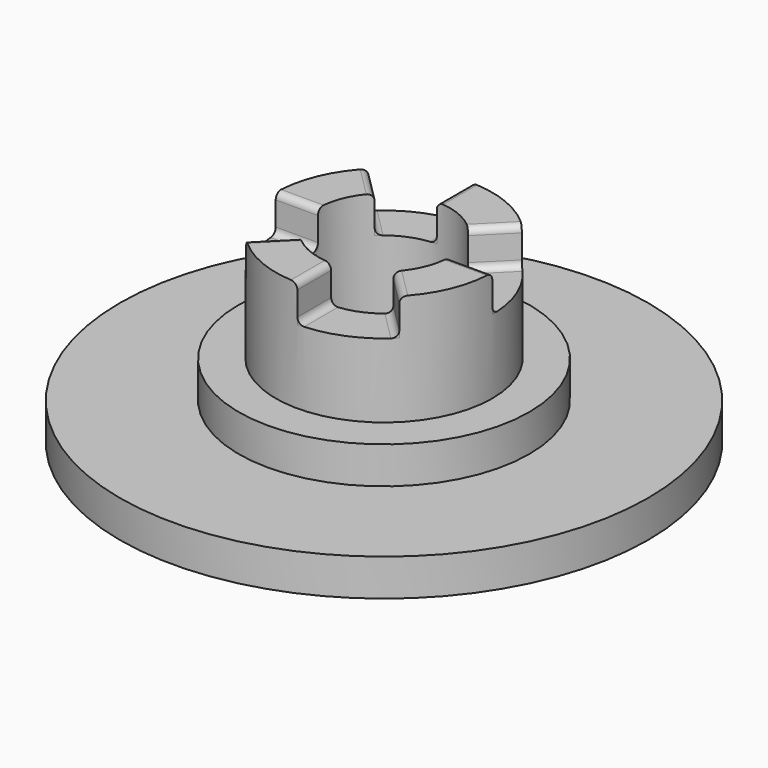
from build123d import *

# Parameters (mm, degrees)
F0_R         = 10
F1_DEPTH     = 1.4
F2_R         = 5.5
F3_DEPTH     = 1.4
F4_R         = 4.1
F4_R_2       = 2.5
F5_DEPTH     = 4.2
F7_DEPTH     = 1.4
F8_T4_DEPTH  = 2.85
F8_S5_R      = 4.1
F8_T6_DEPTH  = 3
F8_S7_R      = 2.5
F8_T8_DEPTH  = 3
F8_T12_DEPTH = 2.85
F8_S13_R     = 4.1
F8_T14_DEPTH = 3
F8_S15_R     = 2.5
F8_T16_DEPTH = 3
F8_T20_DEPTH = 2.85
F8_S21_R     = 4.1
F8_T22_DEPTH = 3
F8_S23_R     = 2.5
F8_T24_DEPTH = 3
F8_T28_DEPTH = 2.85
F8_S29_R     = 4.1
F8_T30_DEPTH = 3
F8_S31_R     = 2.5
F8_T32_DEPTH = 3
F8_T36_DEPTH = 2.85
F8_S37_R     = 4.1
F8_T38_DEPTH = 3
F8_S39_R     = 2.5
F8_T40_DEPTH = 3
F8_T44_DEPTH = 2.85
F8_S45_R     = 4.1
F8_T46_DEPTH = 3
F8_S47_R     = 2.5
F8_T48_DEPTH = 3
F8_T52_DEPTH = 2.85
F8_S53_R     = 4.1
F8_T54_DEPTH = 3
F8_S55_R     = 2.5
F8_T56_DEPTH = 3
F8_T60_DEPTH = 2.85
F8_S61_R     = 4.1
F8_T62_DEPTH = 3
F8_S63_R     = 2.5
F8_T64_DEPTH = 3
F8_T65_DEPTH = 2.85
F8_T67_DEPTH = 2.85
F8_T69_DEPTH = 2.85
F8_T71_DEPTH = 2.85
F8_T73_DEPTH = 2.85
F8_T75_DEPTH = 2.85
F8_T77_DEPTH = 2.85
F8_T79_DEPTH = 2.85


# Not quite as in the source:
# - a fillet or chamfer that OpenCascade refuses, or shapes differently, is made with other operations: its cross-section is extruded or revolved along the edge and cut away or added


with BuildPart() as f1:
    # F0 (on Top) → F1 (new body)
    with BuildSketch(Plane.XY):
        Circle(F0_R)
    extrude(amount=F1_DEPTH)

    # F2 (on face) → F3 (join)
    with BuildSketch(Plane.XY.offset(1.4)):
        Circle(F2_R)
    extrude(amount=F3_DEPTH)

    # F4 (on face) → F5 (join)
    with BuildSketch(Plane.XY.offset(2.8)):
        Circle(F4_R)
        Circle(F4_R_2, mode=Mode.SUBTRACT)
    extrude(amount=F5_DEPTH)

    # F6 (on face) → F7 (cut)
    with BuildSketch(Plane.XY.offset(7)):
        with BuildLine():
            Line((0, -2.5), (0, -4.1))
            ThreePointArc((0, -4.1), (1.5690020727, -3.7879060833), (2.8991378029, -2.8991378029))
            Line((2.8991378029, -2.8991378029), (1.767766953, -1.767766953))
            ThreePointArc((1.767766953, -1.767766953), (0.9567085809, -2.3096988313), (0, -2.5))
        make_face()
        with BuildLine():
            ThreePointArc((-4.1, 0), (-3.7879060833, -1.5690020727), (-2.8991378029, -2.8991378029))
            Line((-2.8991378029, -2.8991378029), (-1.767766953, -1.767766953))
            ThreePointArc((-1.767766953, -1.767766953), (-2.3096988313, -0.9567085809), (-2.5, 0))
            Line((-2.5, 0), (-4.1, 0))
        make_face()
        with BuildLine():
            Line((2.5, 0), (4.1, 0))
            ThreePointArc((4.1, 0), (3.7879060833, 1.5690020727), (2.8991378029, 2.8991378029))
            Line((2.8991378029, 2.8991378029), (1.767766953, 1.767766953))
            ThreePointArc((1.767766953, 1.767766953), (2.3096988313, 0.9567085809), (2.5, 0))
        make_face()
        with BuildLine():
            ThreePointArc((-1.767766953, 1.767766953), (-0.9567085809, 2.3096988313), (0, 2.5))
            Line((0, 2.5), (0, 4.1))
            ThreePointArc((0, 4.1), (-1.5690020727, 3.7879060833), (-2.8991378029, 2.8991378029))
            Line((-2.8991378029, 2.8991378029), (-1.767766953, 1.767766953))
        make_face()
    extrude(amount=-F7_DEPTH, mode=Mode.SUBTRACT)

    # F8: fillet of radius 0.25 on 16 edges, made by hand


with BuildPart() as f8_tool2:
    # F8_s3 → F8_t4 (new body)
    with BuildSketch(Plane.YZ.offset(-1.875)):
        with BuildLine():
            ThreePointArc((-0.25, 5.6), (-0.0732233047, 5.6732233047), (0, 5.85))
            Line((0, 5.85), (0, 5.6))
            Line((0, 5.6), (-0.25, 5.6))
        make_face()
    extrude(amount=-F8_T4_DEPTH)

    # F8_s5 → F8_t6 (intersect, symmetric)
    with BuildSketch(Plane.XY.offset(5.7)):
        Circle(F8_S5_R)
    extrude(amount=F8_T6_DEPTH, both=True, mode=Mode.INTERSECT)

    # F8_s7 → F8_t8 (cut, symmetric)
    with BuildSketch(Plane.XY.offset(5.7)):
        Circle(F8_S7_R)
    extrude(amount=F8_T8_DEPTH, both=True, mode=Mode.SUBTRACT)


with BuildPart() as f1_1:
    add(f1.part)

    # F8_t1: union F8_tool2
    add(f8_tool2.part)


with BuildPart() as f8_tool10:
    # F8_s11 → F8_t12 (new body)
    with BuildSketch(Plane.XZ.offset(-1.875)):
        with BuildLine():
            ThreePointArc((-0.25, 5.6), (-0.0732233047, 5.6732233047), (0, 5.85))
            Line((0, 5.85), (0, 5.6))
            Line((0, 5.6), (-0.25, 5.6))
        make_face()
    extrude(amount=-F8_T12_DEPTH)

    # F8_s13 → F8_t14 (intersect, symmetric)
    with BuildSketch(Plane.XY.offset(5.7)):
        Circle(F8_S13_R)
    extrude(amount=F8_T14_DEPTH, both=True, mode=Mode.INTERSECT)

    # F8_s15 → F8_t16 (cut, symmetric)
    with BuildSketch(Plane.XY.offset(5.7)):
        Circle(F8_S15_R)
    extrude(amount=F8_T16_DEPTH, both=True, mode=Mode.SUBTRACT)


with BuildPart() as f1_2:
    add(f1_1.part)

    # F8_t9: union F8_tool10
    add(f8_tool10.part)


with BuildPart() as f8_tool18:
    # F8_s19 → F8_t20 (new body)
    with BuildSketch(Plane(origin=(3.3410795411, -3.3410795411, 0), x_dir=(0, 0, 1), z_dir=(-0.7071067812, 0.7071067812, 0))):
        with BuildLine():
            ThreePointArc((5.85, 0), (5.6732233047, -0.0732233047), (5.6, -0.25))
            Line((5.6, -0.25), (5.6, 0))
            Line((5.6, 0), (5.85, 0))
        make_face()
    extrude(amount=F8_T20_DEPTH)

    # F8_s21 → F8_t22 (intersect, symmetric)
    with BuildSketch(Plane.XY.offset(5.7)):
        Circle(F8_S21_R)
    extrude(amount=F8_T22_DEPTH, both=True, mode=Mode.INTERSECT)

    # F8_s23 → F8_t24 (cut, symmetric)
    with BuildSketch(Plane.XY.offset(5.7)):
        Circle(F8_S23_R)
    extrude(amount=F8_T24_DEPTH, both=True, mode=Mode.SUBTRACT)


with BuildPart() as f1_3:
    add(f1_2.part)

    # F8_t17: union F8_tool18
    add(f8_tool18.part)


with BuildPart() as f8_tool26:
    # F8_s27 → F8_t28 (new body)
    with BuildSketch(Plane.YZ.offset(1.875)):
        with BuildLine():
            ThreePointArc((0, 5.85), (0.0732233047, 5.6732233047), (0.25, 5.6))
            Line((0.25, 5.6), (0, 5.6))
            Line((0, 5.6), (0, 5.85))
        make_face()
    extrude(amount=F8_T28_DEPTH)

    # F8_s29 → F8_t30 (intersect, symmetric)
    with BuildSketch(Plane.XY.offset(5.7)):
        Circle(F8_S29_R)
    extrude(amount=F8_T30_DEPTH, both=True, mode=Mode.INTERSECT)

    # F8_s31 → F8_t32 (cut, symmetric)
    with BuildSketch(Plane.XY.offset(5.7)):
        Circle(F8_S31_R)
    extrude(amount=F8_T32_DEPTH, both=True, mode=Mode.SUBTRACT)


with BuildPart() as f1_4:
    add(f1_3.part)

    # F8_t25: union F8_tool26
    add(f8_tool26.part)


with BuildPart() as f8_tool34:
    # F8_s35 → F8_t36 (new body)
    with BuildSketch(Plane(origin=(-3.3410795411, -3.3410795411, 0), x_dir=(0, 0, 1), z_dir=(0.7071067812, 0.7071067812, 0))):
        with BuildLine():
            ThreePointArc((5.85, 0), (5.6732233047, -0.0732233047), (5.6, -0.25))
            Line((5.6, -0.25), (5.6, 0))
            Line((5.6, 0), (5.85, 0))
        make_face()
    extrude(amount=F8_T36_DEPTH)

    # F8_s37 → F8_t38 (intersect, symmetric)
    with BuildSketch(Plane.XY.offset(5.7)):
        Circle(F8_S37_R)
    extrude(amount=F8_T38_DEPTH, both=True, mode=Mode.INTERSECT)

    # F8_s39 → F8_t40 (cut, symmetric)
    with BuildSketch(Plane.XY.offset(5.7)):
        Circle(F8_S39_R)
    extrude(amount=F8_T40_DEPTH, both=True, mode=Mode.SUBTRACT)


with BuildPart() as f1_5:
    add(f1_4.part)

    # F8_t33: union F8_tool34
    add(f8_tool34.part)


with BuildPart() as f8_tool42:
    # F8_s43 → F8_t44 (new body)
    with BuildSketch(Plane(origin=(-3.3410795411, 3.3410795411, 0), x_dir=(0, 0, 1), z_dir=(0.7071067812, -0.7071067812, 0))):
        with BuildLine():
            ThreePointArc((5.85, 0), (5.6732233047, -0.0732233047), (5.6, -0.25))
            Line((5.6, -0.25), (5.6, 0))
            Line((5.6, 0), (5.85, 0))
        make_face()
    extrude(amount=F8_T44_DEPTH)

    # F8_s45 → F8_t46 (intersect, symmetric)
    with BuildSketch(Plane.XY.offset(5.7)):
        Circle(F8_S45_R)
    extrude(amount=F8_T46_DEPTH, both=True, mode=Mode.INTERSECT)

    # F8_s47 → F8_t48 (cut, symmetric)
    with BuildSketch(Plane.XY.offset(5.7)):
        Circle(F8_S47_R)
    extrude(amount=F8_T48_DEPTH, both=True, mode=Mode.SUBTRACT)


with BuildPart() as f1_6:
    add(f1_5.part)

    # F8_t41: union F8_tool42
    add(f8_tool42.part)


with BuildPart() as f8_tool50:
    # F8_s51 → F8_t52 (new body)
    with BuildSketch(Plane.XZ.offset(1.875)):
        with BuildLine():
            ThreePointArc((0.25, 5.6), (0.0732233047, 5.6732233047), (0, 5.85))
            Line((0, 5.85), (0, 5.6))
            Line((0, 5.6), (0.25, 5.6))
        make_face()
    extrude(amount=F8_T52_DEPTH)

    # F8_s53 → F8_t54 (intersect, symmetric)
    with BuildSketch(Plane.XY.offset(5.7)):
        Circle(F8_S53_R)
    extrude(amount=F8_T54_DEPTH, both=True, mode=Mode.INTERSECT)

    # F8_s55 → F8_t56 (cut, symmetric)
    with BuildSketch(Plane.XY.offset(5.7)):
        Circle(F8_S55_R)
    extrude(amount=F8_T56_DEPTH, both=True, mode=Mode.SUBTRACT)


with BuildPart() as f1_7:
    add(f1_6.part)

    # F8_t49: union F8_tool50
    add(f8_tool50.part)


with BuildPart() as f8_tool58:
    # F8_s59 → F8_t60 (new body)
    with BuildSketch(Plane(origin=(3.3410795411, 3.3410795411, 0), x_dir=(0, 0, 1), z_dir=(-0.7071067812, -0.7071067812, 0))):
        with BuildLine():
            ThreePointArc((5.85, 0), (5.6732233047, -0.0732233047), (5.6, -0.25))
            Line((5.6, -0.25), (5.6, 0))
            Line((5.6, 0), (5.85, 0))
        make_face()
    extrude(amount=F8_T60_DEPTH)

    # F8_s61 → F8_t62 (intersect, symmetric)
    with BuildSketch(Plane.XY.offset(5.7)):
        Circle(F8_S61_R)
    extrude(amount=F8_T62_DEPTH, both=True, mode=Mode.INTERSECT)

    # F8_s63 → F8_t64 (cut, symmetric)
    with BuildSketch(Plane.XY.offset(5.7)):
        Circle(F8_S63_R)
    extrude(amount=F8_T64_DEPTH, both=True, mode=Mode.SUBTRACT)


with BuildPart() as f1_8:
    add(f1_7.part)

    # F8_t57: union F8_tool58
    add(f8_tool58.part)

    # F8_s66 → F8_t65 (cut)
    with BuildSketch(Plane.YZ.offset(-4.725)):
        with BuildLine():
            ThreePointArc((0, 6.75), (0.0732233047, 6.9267766953), (0.25, 7))
            Line((0.25, 7), (0, 7))
            Line((0, 7), (0, 6.75))
        make_face()
    extrude(amount=F8_T65_DEPTH, mode=Mode.SUBTRACT)

    # F8_s68 → F8_t67 (cut)
    with BuildSketch(Plane(origin=(-3.3410795411, 3.3410795411, 0), x_dir=(0, 0, 1), z_dir=(0.7071067812, -0.7071067812, 0))):
        with BuildLine():
            ThreePointArc((7, 0.25), (6.9267766953, 0.0732233047), (6.75, 0))
            Line((6.75, 0), (7, 0))
            Line((7, 0), (7, 0.25))
        make_face()
    extrude(amount=F8_T67_DEPTH, mode=Mode.SUBTRACT)

    # F8_s70 → F8_t69 (cut)
    with BuildSketch(Plane.XZ.offset(1.875)):
        with BuildLine():
            ThreePointArc((0, 6.75), (-0.0732233047, 6.9267766953), (-0.25, 7))
            Line((-0.25, 7), (0, 7))
            Line((0, 7), (0, 6.75))
        make_face()
    extrude(amount=F8_T69_DEPTH, mode=Mode.SUBTRACT)

    # F8_s72 → F8_t71 (cut)
    with BuildSketch(Plane(origin=(-3.3410795411, -3.3410795411, 0), x_dir=(0, 0, 1), z_dir=(0.7071067812, 0.7071067812, 0))):
        with BuildLine():
            ThreePointArc((7, 0.25), (6.9267766953, 0.0732233047), (6.75, 0))
            Line((6.75, 0), (7, 0))
            Line((7, 0), (7, 0.25))
        make_face()
    extrude(amount=F8_T71_DEPTH, mode=Mode.SUBTRACT)

    # F8_s74 → F8_t73 (cut)
    with BuildSketch(Plane.YZ.offset(1.875)):
        with BuildLine():
            ThreePointArc((0, 6.75), (-0.0732233047, 6.9267766953), (-0.25, 7))
            Line((-0.25, 7), (0, 7))
            Line((0, 7), (0, 6.75))
        make_face()
    extrude(amount=F8_T73_DEPTH, mode=Mode.SUBTRACT)

    # F8_s76 → F8_t75 (cut)
    with BuildSketch(Plane(origin=(3.3410795411, -3.3410795411, 0), x_dir=(0, 0, 1), z_dir=(-0.7071067812, 0.7071067812, 0))):
        with BuildLine():
            ThreePointArc((7, 0.25), (6.9267766953, 0.0732233047), (6.75, 0))
            Line((6.75, 0), (7, 0))
            Line((7, 0), (7, 0.25))
        make_face()
    extrude(amount=F8_T75_DEPTH, mode=Mode.SUBTRACT)

    # F8_s78 → F8_t77 (cut)
    with BuildSketch(Plane.XZ.offset(-4.725)):
        with BuildLine():
            ThreePointArc((0, 6.75), (0.0732233047, 6.9267766953), (0.25, 7))
            Line((0.25, 7), (0, 7))
            Line((0, 7), (0, 6.75))
        make_face()
    extrude(amount=F8_T77_DEPTH, mode=Mode.SUBTRACT)

    # F8_s80 → F8_t79 (cut)
    with BuildSketch(Plane(origin=(3.3410795411, 3.3410795411, 0), x_dir=(0, 0, 1), z_dir=(-0.7071067812, -0.7071067812, 0))):
        with BuildLine():
            ThreePointArc((7, 0.25), (6.9267766953, 0.0732233047), (6.75, 0))
            Line((6.75, 0), (7, 0))
            Line((7, 0), (7, 0.25))
        make_face()
    extrude(amount=F8_T79_DEPTH, mode=Mode.SUBTRACT)


solid = f1_8.part
